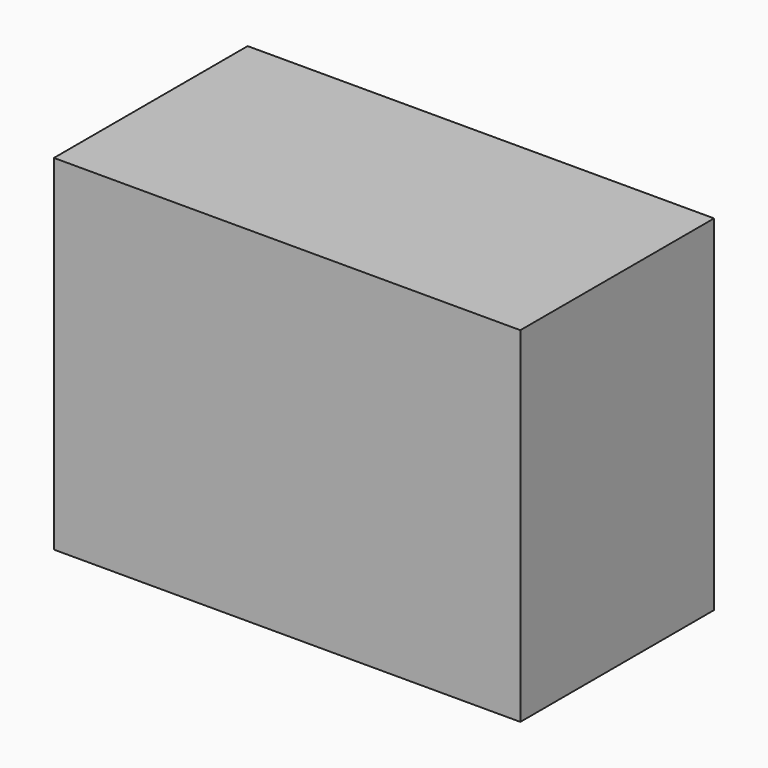
from build123d import *

# Parameters (mm, degrees)
F5_W     = 57.1044310927
F5_H     = 81.3167020679
F6_DEPTH = 109.982


# Not quite as in the source:
# - the program builds the solid bodies; features that only make, move or delete a surface that nothing else refers to are left out


with BuildPart() as f6:
    # F5 (on Right) → F6 (new body)
    with BuildSketch(Plane.YZ):
        with Locations((151.6078449786, 66.3434751332)):
            Rectangle(F5_W, F5_H)
    extrude(amount=-F6_DEPTH)


solid = f6.part
